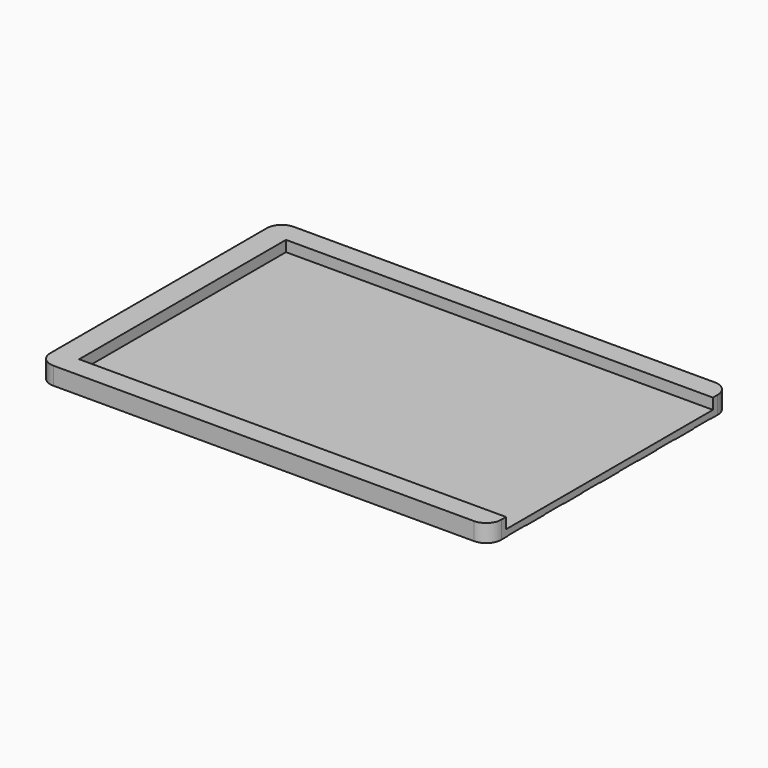
from build123d import *

# Parameters (mm, degrees)
F1_DEPTH = 3.7338
F2_W     = 90.17
F2_H     = 54.61
F3_DEPTH = 2.286
F4_W     = 55.5096130292
F4_H     = 4.9022
F4_W_2   = 95.25
F4_H_2   = 4.6736
F5_DEPTH = 0.0762


with BuildPart() as f1:
    # F0 (on Top) → F1 (new body)
    with BuildSketch(Plane.XY):
        with BuildLine():
            Line((-44.45, -31.75), (44.45, -31.75))
            ThreePointArc((44.45, -31.75), (46.6950640303, -30.8200640303), (47.625, -28.575))
            Line((47.625, -28.575), (47.625, 28.575))
            ThreePointArc((47.625, 28.575), (46.6950640303, 30.8200640303), (44.45, 31.75))
            Line((44.45, 31.75), (-44.45, 31.75))
            ThreePointArc((-44.45, 31.75), (-46.6950640303, 30.8200640303), (-47.625, 28.575))
            Line((-47.625, 28.575), (-47.625, -28.575))
            ThreePointArc((-47.625, -28.575), (-46.6950640303, -30.8200640303), (-44.45, -31.75))
        make_face()
    extrude(amount=F1_DEPTH)

    # F2 (on face) → F3 (cut)
    with BuildSketch(Plane.XY.offset(3.7338)):
        with Locations((2.54, 0)):
            Rectangle(F2_W, F2_H)
    extrude(amount=-F3_DEPTH, mode=Mode.SUBTRACT)

    # F4 (on face) → F5 (cut)
    with BuildSketch(Plane(origin=(0, 0, 0), x_dir=(1, 0, 0), z_dir=(0, 0, -1))):
        with Locations((19.8701934854, 24.3967)):
            Rectangle(F4_W, F4_H)
        with Locations((19.8701934854, 14.5923)):
            Rectangle(F4_W, F4_H)
        with Locations((19.8701934854, 4.7879)):
            Rectangle(F4_W, F4_H)
        with Locations((0, -5.0165)):
            Rectangle(F4_W_2, F4_H)
        with Locations((0, -14.8209)):
            Rectangle(F4_W_2, F4_H)
        with Locations((0, -24.511)):
            Rectangle(F4_W_2, F4_H_2)
        Polygon((-45.1385900378, 29.5881610364), (-45.9221303463, 29.5881610364), (-45.2595762908, 29.0120523423), (-45.3805625439, 28.2285436988), (-44.6719229221, 28.6145377904), (-44.0554618835, 28.2285436988), (-44.2283004522, 29.0639027953), (-43.6521694064, 29.5881610364), (-44.4414690137, 29.5881610364), (-44.7986721992, 30.3025357425), align=None)
        Polygon((-38.0548011512, 29.5662444085), (-38.8383414596, 29.5662444085), (-38.1757874042, 28.9901357144), (-38.2967736572, 28.2066270709), (-37.5881340355, 28.5926211625), (-36.9716729969, 28.2066270709), (-37.1445115656, 29.0419861674), (-36.5683805197, 29.5662444085), (-37.357680127, 29.5662444085), (-37.7148833126, 30.2806191146), align=None)
        Polygon((-20.7016129047, 6.4387788996), (-21.4851532131, 6.4387788996), (-20.8225991577, 5.8626702055), (-20.9435854107, 5.079161562), (-20.234945789, 5.4651556537), (-19.6184847504, 5.079161562), (-19.7913233191, 5.9145206586), (-19.2151922733, 6.4387788996), (-20.0044918805, 6.4387788996), (-20.3616950661, 7.1531536058), align=None)
        Polygon((-17.1554531902, 3.5707323812), (-17.9389934987, 3.5707323812), (-17.2764394432, 2.9946236871), (-17.3974256963, 2.2111150436), (-16.6887860745, 2.5971091352), (-16.0723250359, 2.2111150436), (-16.2451636046, 3.0464741401), (-15.6690325588, 3.5707323812), (-16.4583321661, 3.5707323812), (-16.8155353516, 4.2851070873), align=None)
        Polygon((-13.648051396, 6.5744297579), (-14.4315917045, 6.5744297579), (-13.769037649, 5.9983210638), (-13.8900239021, 5.2148124203), (-13.1813842803, 5.6008065119), (-12.5649232417, 5.2148124203), (-12.7377618104, 6.0501715168), (-12.1616307646, 6.5744297579), (-12.9509303719, 6.5744297579), (-13.3081335574, 7.288804464), align=None)
        Polygon((-10.1600266993, 3.5319751594), (-10.9435670078, 3.5319751594), (-10.2810129523, 2.9558664653), (-10.4019992054, 2.1723578218), (-9.6933595836, 2.5583519135), (-9.076898545, 2.1723578218), (-9.2497371137, 3.0077169184), (-8.6736060679, 3.5319751594), (-9.4629056752, 3.5319751594), (-9.8201088607, 4.2463498656), align=None)
        Polygon((-10.1406486705, 10.0819721818), (-10.924188979, 10.0819721818), (-10.2616349235, 9.5058634877), (-10.3826211765, 8.7223548442), (-9.6739815548, 9.1083489358), (-9.0575205162, 8.7223548442), (-9.2303590849, 9.5577139407), (-8.6542280391, 10.0819721818), (-9.4435276464, 10.0819721818), (-9.8007308319, 10.7963468879), align=None)
        Polygon((-17.1748321503, 9.9463222548), (-17.9583724588, 9.9463222548), (-17.2958184034, 9.3702135608), (-17.4168046564, 8.5867049173), (-16.7081650347, 8.9726990089), (-16.0917039961, 8.5867049173), (-16.2645425647, 9.4220640138), (-15.6884115189, 9.9463222548), (-16.4777111262, 9.9463222548), (-16.8349143118, 10.660696961), align=None)
        Polygon((-24.1508815438, 3.6676260177), (-24.9344218522, 3.6676260177), (-24.2718677968, 3.0915173236), (-24.3928540498, 2.3080086801), (-23.6842144281, 2.6940027718), (-23.0677533895, 2.3080086801), (-23.2405919582, 3.1433677766), (-22.6644609123, 3.6676260177), (-23.4537605196, 3.6676260177), (-23.8109637052, 4.3820007239), align=None)
        Polygon((-41.5216419846, 26.2572217733), (-42.3051822931, 26.2572217733), (-41.6426282376, 25.6811130792), (-41.7636144906, 24.8976044357), (-41.0549748689, 25.2835985273), (-40.4385138303, 24.8976044357), (-40.611352399, 25.7329635322), (-40.0352213532, 26.2572217733), (-40.8245209605, 26.2572217733), (-41.181724146, 26.9715964794), align=None)
        Polygon((-45.0484227389, 23.2730221003), (-45.8319630474, 23.2730221003), (-45.1694089919, 22.6969134063), (-45.290395245, 21.9134047627), (-44.5817556232, 22.2993988544), (-43.9652945846, 21.9134047627), (-44.1381331533, 22.7487638593), (-43.5620021075, 23.2730221003), (-44.3513017148, 23.2730221003), (-44.7085049003, 23.9873968065), align=None)
        Polygon((-38.1498854607, 23.1567539275), (-38.9334257692, 23.1567539275), (-38.2708717138, 22.5806452334), (-38.3918579668, 21.7971365899), (-37.683218345, 22.1831306815), (-37.0667573065, 21.7971365899), (-37.2395958751, 22.6324956864), (-36.6634648293, 23.1567539275), (-37.4527644366, 23.1567539275), (-37.8099676222, 23.8711286336), align=None)
        Polygon((-34.5843505114, 26.2572217733), (-35.3678908199, 26.2572217733), (-34.7053367645, 25.6811130792), (-34.8263230175, 24.8976044357), (-34.1176833957, 25.2835985273), (-33.5012223572, 24.8976044357), (-33.6740609258, 25.7329635322), (-33.09792988, 26.2572217733), (-33.8872294873, 26.2572217733), (-34.2444326729, 26.9715964794), align=None)
        Polygon((-31.1738360673, 29.5127101243), (-31.9573763758, 29.5127101243), (-31.2948223203, 28.9366014302), (-31.4158085734, 28.1530927867), (-30.7071689516, 28.5390868783), (-30.090707913, 28.1530927867), (-30.2635464817, 28.9884518832), (-29.6874154359, 29.5127101243), (-30.4767150432, 29.5127101243), (-30.8339182287, 30.2270848304), align=None)
        Polygon((-27.5695431978, 26.1409536004), (-28.3530835062, 26.1409536004), (-27.6905294508, 25.5648449063), (-27.8115157038, 24.7813362628), (-27.1028760821, 25.1673303545), (-26.4864150435, 24.7813362628), (-26.6592536122, 25.6166953593), (-26.0831225663, 26.1409536004), (-26.8724221736, 26.1409536004), (-27.2296253592, 26.8553283066), align=None)
        Polygon((-23.9652521908, 29.6289782971), (-24.7487924993, 29.6289782971), (-24.0862384439, 29.052869603), (-24.2072246969, 28.2693609595), (-23.4985850751, 28.6553550512), (-22.8821240366, 28.2693609595), (-23.0549626052, 29.1047200561), (-22.4788315594, 29.6289782971), (-23.2681311667, 29.6289782971), (-23.6253343523, 30.3433530033), align=None)
        Polygon((-20.5547396094, 26.179709658), (-21.3382799178, 26.179709658), (-20.6757258624, 25.603600964), (-20.7967121154, 24.8200923204), (-20.0880724937, 25.2060864121), (-19.4716114551, 24.8200923204), (-19.6444500238, 25.655451417), (-19.068318978, 26.179709658), (-19.8576185852, 26.179709658), (-20.2148217708, 26.8940843642), align=None)
        Polygon((-17.1054709703, 29.5127101243), (-17.8890112787, 29.5127101243), (-17.2264572233, 28.9366014302), (-17.3474434763, 28.1530927867), (-16.6388038546, 28.5390868783), (-16.022342816, 28.1530927867), (-16.1951813847, 28.9884518832), (-15.6190503389, 29.5127101243), (-16.4083499461, 29.5127101243), (-16.7655531317, 30.2270848304), align=None)
        Polygon((-13.6562013999, 26.3347338885), (-14.4397417083, 26.3347338885), (-13.7771876529, 25.7586251944), (-13.8981739059, 24.9751165509), (-13.1895342842, 25.3611106426), (-12.5730732456, 24.9751165509), (-12.7459118143, 25.8104756474), (-12.1697807685, 26.3347338885), (-12.9590803757, 26.3347338885), (-13.3162835613, 27.0491085947), align=None)
        Polygon((-10.1681767032, 29.6291105449), (-10.9517170116, 29.6291105449), (-10.2891629562, 29.0530018508), (-10.4101492092, 28.2694932073), (-9.7015095875, 28.655487299), (-9.0850485489, 28.2694932073), (-9.2578871176, 29.1048523039), (-8.6817560717, 29.6291105449), (-9.471055679, 29.6291105449), (-9.8282588646, 30.3434852511), align=None)
        Polygon((-10.1294206455, 23.2729010284), (-10.912960954, 23.2729010284), (-10.2504068986, 22.6967923343), (-10.3713931516, 21.9132836908), (-9.6627535298, 22.2992777824), (-9.0462924913, 21.9132836908), (-9.2191310599, 22.7486427873), (-8.6430000141, 23.2729010284), (-9.4322996214, 23.2729010284), (-9.789502807, 23.9872757345), align=None)
        Polygon((-17.1442251652, 23.2729010284), (-17.9277654737, 23.2729010284), (-17.2652114183, 22.6967923343), (-17.3861976713, 21.9132836908), (-16.6775580496, 22.2992777824), (-16.061097011, 21.9132836908), (-16.2339355797, 22.7486427873), (-15.6578045338, 23.2729010284), (-16.4471041411, 23.2729010284), (-16.8043073267, 23.9872757345), align=None)
        Polygon((-24.1590306163, 23.3116589487), (-24.9425709248, 23.3116589487), (-24.2800168693, 22.7355502546), (-24.4010031223, 21.9520416111), (-23.6923635006, 22.3380357027), (-23.075902462, 21.9520416111), (-23.2487410307, 22.7874007076), (-22.6726099849, 23.3116589487), (-23.4619095922, 23.3116589487), (-23.8191127777, 24.0260336548), align=None)
        Polygon((-31.2125921249, 23.3504150063), (-31.9961324334, 23.3504150063), (-31.333578378, 22.7743063122), (-31.454564631, 21.9907976687), (-30.7459250093, 22.3767917603), (-30.1294639707, 21.9907976687), (-30.3023025393, 22.8261567652), (-29.7261714935, 23.3504150063), (-30.5154711008, 23.3504150063), (-30.8726742864, 24.0647897124), align=None)
        Polygon((-41.6379120201, 19.9010085315), (-42.4214523286, 19.9010085315), (-41.7588982731, 19.3248998374), (-41.8798845261, 18.5413911939), (-41.1712449044, 18.9273852855), (-40.5547838658, 18.5413911939), (-40.7276224345, 19.3767502904), (-40.1514913887, 19.9010085315), (-40.940790996, 19.9010085315), (-41.2979941815, 20.6153832376), align=None)
        Polygon((-34.4680842012, 19.745978713), (-35.2516245097, 19.745978713), (-34.5890704542, 19.169870019), (-34.7100567073, 18.3863613755), (-34.0014170855, 18.7723554671), (-33.3849560469, 18.3863613755), (-33.5577946156, 19.221720472), (-32.9816635698, 19.745978713), (-33.7709631771, 19.745978713), (-34.1281663626, 20.4603534192), align=None)
        Polygon((-27.5307890028, 19.8622506112), (-28.3143293113, 19.8622506112), (-27.6517752558, 19.2861419171), (-27.7727615088, 18.5026332736), (-27.0641218871, 18.8886273652), (-26.4476608485, 18.5026332736), (-26.6204994172, 19.3379923701), (-26.0443683714, 19.8622506112), (-26.8336679786, 19.8622506112), (-27.1908711642, 20.5766253173), align=None)
        Polygon((-20.4772274941, 19.8622506112), (-21.2607678026, 19.8622506112), (-20.5982137471, 19.2861419171), (-20.7192000002, 18.5026332736), (-20.0105603784, 18.8886273652), (-19.3940993398, 18.5026332736), (-19.5669379085, 19.3379923701), (-18.9908068627, 19.8622506112), (-19.78010647, 19.8622506112), (-20.1373096555, 20.5766253173), align=None)
        Polygon((-13.6949565262, 19.745978713), (-14.4784968346, 19.745978713), (-13.8159427792, 19.169870019), (-13.9369290322, 18.3863613755), (-13.2282894105, 18.7723554671), (-12.6118283719, 18.3863613755), (-12.7846669406, 19.221720472), (-12.2085358948, 19.745978713), (-12.997835502, 19.745978713), (-13.3550386876, 20.4603534192), align=None)
        Polygon((-10.1294206455, 16.6841458529), (-10.912960954, 16.6841458529), (-10.2504068986, 16.1080371588), (-10.3713931516, 15.3245285153), (-9.6627535298, 15.710522607), (-9.0462924913, 15.3245285153), (-9.2191310599, 16.1598876119), (-8.6430000141, 16.6841458529), (-9.4322996214, 16.6841458529), (-9.789502807, 17.3985205591), align=None)
        Polygon((-17.1054709703, 16.606631875), (-17.8890112787, 16.606631875), (-17.2264572233, 16.030523181), (-17.3474434763, 15.2470145375), (-16.6388038546, 15.6330086291), (-16.022342816, 15.2470145375), (-16.1951813847, 16.082373634), (-15.6190503389, 16.606631875), (-16.4083499461, 16.606631875), (-16.7655531317, 17.3210065812), align=None)
        Polygon((-24.1590306163, 16.606631875), (-24.9425709248, 16.606631875), (-24.2800168693, 16.030523181), (-24.4010031223, 15.2470145375), (-23.6923635006, 15.6330086291), (-23.075902462, 15.2470145375), (-23.2487410307, 16.082373634), (-22.6726099849, 16.606631875), (-23.4619095922, 16.606631875), (-23.8191127777, 17.3210065812), align=None)
        Polygon((-31.1738360673, 16.606631875), (-31.9573763758, 16.606631875), (-31.2948223203, 16.030523181), (-31.4158085734, 15.2470145375), (-30.7071689516, 15.6330086291), (-30.090707913, 15.2470145375), (-30.2635464817, 16.082373634), (-29.6874154359, 16.606631875), (-30.4767150432, 16.606631875), (-30.8339182287, 17.3210065812), align=None)
        Polygon((-38.1111312658, 16.5678739548), (-38.8946715742, 16.5678739548), (-38.2321175188, 15.9917652607), (-38.3531037718, 15.2082566172), (-37.6444641501, 15.5942507088), (-37.0280031115, 15.2082566172), (-37.2008416802, 16.0436157137), (-36.6247106344, 16.5678739548), (-37.4140102416, 16.5678739548), (-37.7712134272, 17.2822486609), align=None)
        Polygon((-45.0484227389, 16.6453879327), (-45.8319630474, 16.6453879327), (-45.1694089919, 16.0692792386), (-45.290395245, 15.2857705951), (-44.5817556232, 15.6717646867), (-43.9652945846, 15.2857705951), (-44.1381331533, 16.1211296916), (-43.5620021075, 16.6453879327), (-44.3513017148, 16.6453879327), (-44.7085049003, 17.3597626388), align=None)
        Polygon((-13.6562013999, 13.1572244689), (-14.4397417083, 13.1572244689), (-13.7771876529, 12.5811157748), (-13.8981739059, 11.7976071313), (-13.1895342842, 12.1836012229), (-12.5730732456, 11.7976071313), (-12.7459118143, 12.6329662278), (-12.1697807685, 13.1572244689), (-12.9590803757, 13.1572244689), (-13.3162835613, 13.871599175), align=None)
        Polygon((-20.632249862, 13.1572244689), (-21.4157901704, 13.1572244689), (-20.753236115, 12.5811157748), (-20.874222368, 11.7976071313), (-20.1655827463, 12.1836012229), (-19.5491217077, 11.7976071313), (-19.7219602764, 12.6329662278), (-19.1458292305, 13.1572244689), (-19.9351288378, 13.1572244689), (-20.2923320234, 13.871599175), align=None)
        Polygon((-27.6858113706, 13.1959814578), (-28.4693516791, 13.1959814578), (-27.8067976236, 12.6198727638), (-27.9277838767, 11.8363641202), (-27.2191442549, 12.2223582119), (-26.6026832163, 11.8363641202), (-26.775521785, 12.6717232168), (-26.1993907392, 13.1959814578), (-26.9886903465, 13.1959814578), (-27.345893532, 13.910356164), align=None)
        Polygon((-34.6231047064, 13.1959814578), (-35.4066450149, 13.1959814578), (-34.7440909594, 12.6198727638), (-34.8650772125, 11.8363641202), (-34.1564375907, 12.2223582119), (-33.5399765521, 11.8363641202), (-33.7128151208, 12.6717232168), (-33.136684075, 13.1959814578), (-33.9259836823, 13.1959814578), (-34.2831868678, 13.910356164), align=None)
        Polygon((-41.5991540998, 13.1572244689), (-42.3826944083, 13.1572244689), (-41.7201403528, 12.5811157748), (-41.8411266059, 11.7976071313), (-41.1324869841, 12.1836012229), (-40.5160259455, 11.7976071313), (-40.6888645142, 12.6329662278), (-40.1127334684, 13.1572244689), (-40.9020330757, 13.1572244689), (-41.2592362612, 13.871599175), align=None)
        Polygon((-45.0871806592, 9.8628468812), (-45.8707209677, 9.8628468812), (-45.2081669122, 9.2867381871), (-45.3291531652, 8.5032295436), (-44.6205135435, 8.8892236352), (-44.0040525049, 8.5032295436), (-44.1768910736, 9.3385886401), (-43.6007600278, 9.8628468812), (-44.390059635, 9.8628468812), (-44.7472628206, 10.5772215873), align=None)
        Polygon((-38.1111312658, 10.0178757682), (-38.8946715742, 10.0178757682), (-38.2321175188, 9.4417670742), (-38.3531037718, 8.6582584307), (-37.6444641501, 9.0442525223), (-37.0280031115, 8.6582584307), (-37.2008416802, 9.4936175272), (-36.6247106344, 10.0178757682), (-37.4140102416, 10.0178757682), (-37.7712134272, 10.7322504744), align=None)
        Polygon((-31.0963258147, 9.9016038701), (-31.8798661232, 9.9016038701), (-31.2173120677, 9.325495176), (-31.3382983208, 8.5419865325), (-30.629658699, 8.9279806241), (-30.0131976604, 8.5419865325), (-30.1860362291, 9.377345629), (-29.6099051833, 9.9016038701), (-30.3992047906, 9.9016038701), (-30.7564079762, 10.6159785762), align=None)
        Polygon((-24.081518501, 9.9016038701), (-24.8650588095, 9.9016038701), (-24.2025047541, 9.325495176), (-24.3234910071, 8.5419865325), (-23.6148513854, 8.9279806241), (-22.9983903468, 8.5419865325), (-23.1712289155, 9.377345629), (-22.5950978696, 9.9016038701), (-23.3843974769, 9.9016038701), (-23.7416006625, 10.6159785762), align=None)
        Polygon((-27.608301118, 6.413439475), (-28.3918414265, 6.413439475), (-27.729287371, 5.8373307809), (-27.8502736241, 5.0538221374), (-27.1416340023, 5.439816229), (-26.5251729637, 5.0538221374), (-26.6980115324, 5.8891812339), (-26.1218804866, 6.413439475), (-26.9111800939, 6.413439475), (-27.2683832794, 7.1278141811), align=None)
        Polygon((-34.6231047064, 6.413439475), (-35.4066450149, 6.413439475), (-34.7440909594, 5.8373307809), (-34.8650772125, 5.0538221374), (-34.1564375907, 5.439816229), (-33.5399765521, 5.0538221374), (-33.7128151208, 5.8891812339), (-33.136684075, 6.413439475), (-33.9259836823, 6.413439475), (-34.2831868678, 7.1278141811), align=None)
        Polygon((-41.5603999048, 6.3359250315), (-42.3439402133, 6.3359250315), (-41.6813861579, 5.7598163374), (-41.8023724109, 4.9763076939), (-41.0937327892, 5.3623017855), (-40.4772717506, 4.9763076939), (-40.6501103193, 5.8116667904), (-40.0739792734, 6.3359250315), (-40.8632788807, 6.3359250315), (-41.2204820663, 7.0502997376), align=None)
        Polygon((-45.0484227389, 3.584150644), (-45.8319630474, 3.584150644), (-45.1694089919, 3.0080419499), (-45.290395245, 2.2245333064), (-44.5817556232, 2.6105273981), (-43.9652945846, 2.2245333064), (-44.1381331533, 3.059892403), (-43.5620021075, 3.584150644), (-44.3513017148, 3.584150644), (-44.7085049003, 4.2985253502), align=None)
        Polygon((-38.0336191505, 3.6616648547), (-38.817159459, 3.6616648547), (-38.1546054035, 3.0855561607), (-38.2755916566, 2.3020475172), (-37.5669520348, 2.6880416088), (-36.9504909962, 2.3020475172), (-37.1233295649, 3.1374066137), (-36.5471985191, 3.6616648547), (-37.3364981264, 3.6616648547), (-37.6937013119, 4.3760395609), align=None)
        Polygon((-31.1350818723, 3.584150644), (-31.9186221808, 3.584150644), (-31.2560681254, 3.0080419499), (-31.3770543784, 2.2245333064), (-30.6684147567, 2.6105273981), (-30.0519537181, 2.2245333064), (-30.2247922868, 3.059892403), (-29.6486612409, 3.584150644), (-30.4379608482, 3.584150644), (-30.7951640338, 4.2985253502), align=None)
    extrude(amount=-F5_DEPTH, mode=Mode.SUBTRACT)


solid = f1.part
